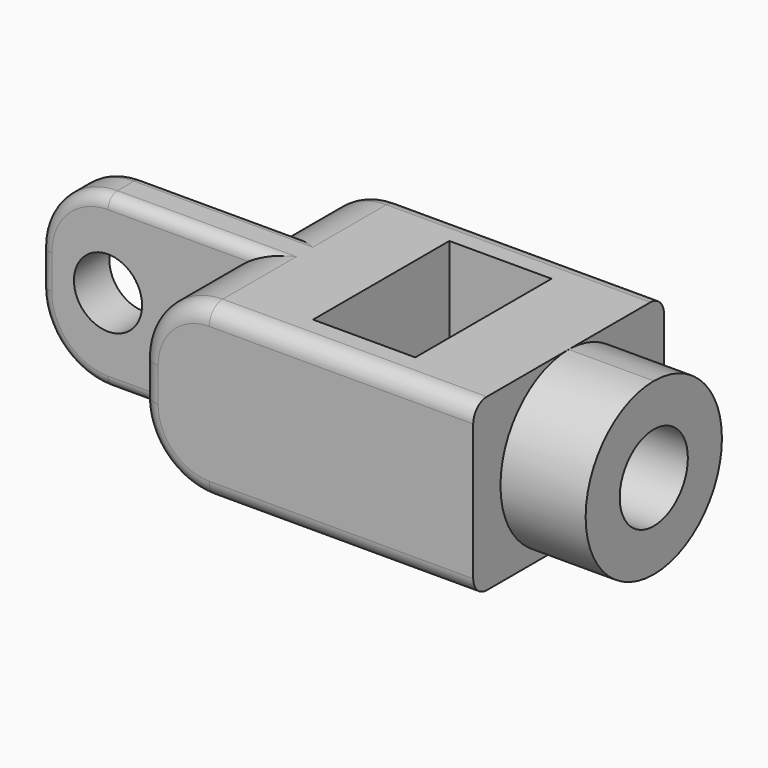
from build123d import *

# Parameters (mm, degrees)
F0_W      = 30
F0_H      = 14
F1_DEPTH  = 10
F2_W      = 10.5
F2_H      = 5.7
F3_DEPTH  = 25
F4_R      = 4
F5_R      = 2
F6_DEPTH  = 25
F8_DEPTH  = 5
F10_DEPTH = 12
F11_R     = 0.7
F12_R     = 1
F13_R     = 2.5
F14_DEPTH = 15


with BuildPart() as f1:
    # F0 (on Top) → F1 (new body)
    with BuildSketch(Plane.XY):
        Rectangle(F0_W, F0_H)
    extrude(amount=F1_DEPTH)

    # F2 (on face) → F3 (cut)
    with BuildSketch(Plane.XY.offset(10)):
        with Locations((-9.75, -4.15)):
            Rectangle(F2_W, F2_H)
        with Locations((-9.75, 4.15)):
            Rectangle(F2_W, F2_H)
    extrude(amount=-F3_DEPTH, mode=Mode.SUBTRACT)

    # F4
    f4_edges = [f1.edges().sort_by_distance(p)[0] for p in [
        (-15, 0, 10),
        (-15, 0, 0),
        (-4.5, -4.15, 10),
        (-4.5, -4.15, 0),
        (-4.5, 4.15, 0),
        (-4.5, 4.15, 10),
    ]]
    fillet(f4_edges, radius=F4_R)

    # F5 (on face) → F6 (cut)
    with BuildSketch(Plane.XZ.offset(1.3)):
        with Locations((-11, 5)):
            Circle(F5_R)
    extrude(amount=-F6_DEPTH, mode=Mode.SUBTRACT)

    # F7 (on face) → F8 (join)
    with BuildSketch(Plane.YZ.offset(15)):
        with BuildLine():
            ThreePointArc((0, 0), (3.5355339059, 1.4644660941), (5, 5))
            ThreePointArc((5, 5), (3.5355339059, 8.5355339059), (0, 10))
            ThreePointArc((0, 10), (-5, 5), (0, 0))
        make_face()
    extrude(amount=F8_DEPTH)

    # F9 (on face) → F10 (cut)
    with BuildSketch(Plane.XY.offset(10)):
        Polygon((10, -5), (9.9985566437, 5), (3.9985566437, 5), (3.9985566437, -5), align=None)
    extrude(amount=-F10_DEPTH, mode=Mode.SUBTRACT)

    # F11
    f11_edges = [f1.edges().sort_by_distance(p)[0] for p in [
        (-5.75, -1.3, 10),
        (-5.75, -1.3, 0),
        (-13.828427, -1.3, 1.171573),
        (-15, -1.3, 5),
        (-13.828427, -1.3, 8.828427),
        (-5.75, 1.3, 0),
        (-13.828427, 1.3, 1.171573),
        (-15, 1.3, 5),
        (-13.828427, 1.3, 8.828427),
        (-5.75, 1.3, 10),
    ]]
    fillet(f11_edges, radius=F11_R)

    # F12
    f12_edges = [f1.edges().sort_by_distance(p)[0] for p in [
        (7.25, -7, 10),
        (-3.328427, -7, 1.171573),
        (-4.5, -7, 5),
        (-3.328427, -7, 8.828427),
        (7.25, 7, 10),
    ]]
    fillet(f12_edges, radius=F12_R)

    # F13 (on face) → F14 (cut)
    with BuildSketch(Plane.YZ.offset(20)):
        with Locations((0, 5)):
            Circle(F13_R)
    extrude(amount=-F14_DEPTH, mode=Mode.SUBTRACT)


solid = f1.part
